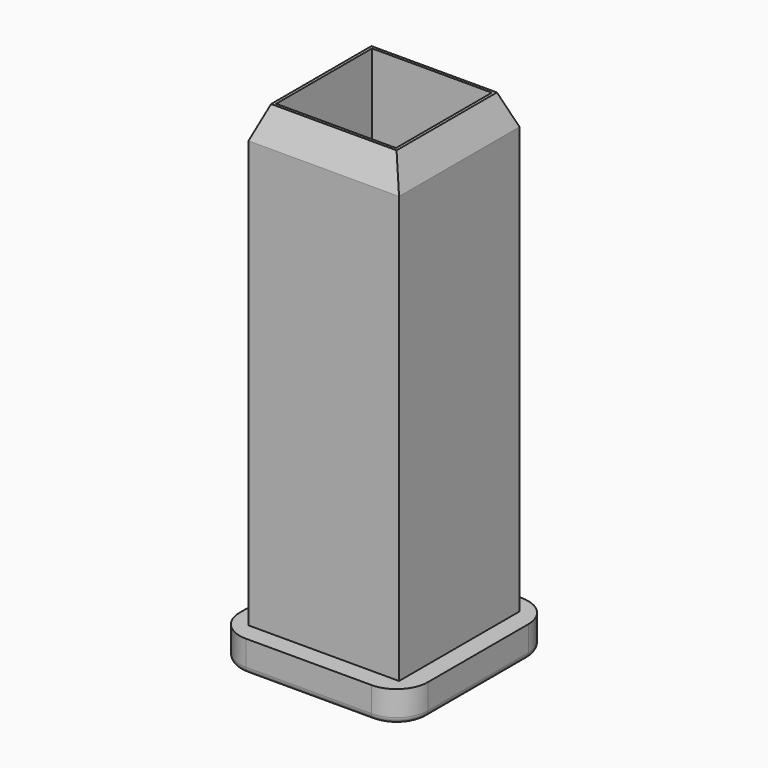
from build123d import *

# Parameters (mm, degrees)
F0_W         = 24
F0_H         = 24
F0_W_2       = 19.1
F0_H_2       = 19.1
F1_DEPTH     = 73
F2_W         = 30
F2_H         = 30
F2_W_2       = 19.1615689546
F2_H_2       = 19.1443199292
F3_DEPTH     = 5
F4_T4_DEPTH  = 19.1615689546
F4_T9_DEPTH  = 19.1443199292
F4_T14_DEPTH = 19.1615689546
F4_T19_DEPTH = 19.1443199292
F4_T25_DEPTH = 45.1428898176
F4_T30_DEPTH = 45.1256407922
F4_T38_DEPTH = 45.1428898176
F4_T43_DEPTH = 45.1256407922
F4_T51_DEPTH = 45.1428898176
F4_T56_DEPTH = 45.1256407922
F4_T64_DEPTH = 45.1256407922
F4_T69_DEPTH = 45.1428898176
F5_SIZE2     = 3
F5_SIZE      = 1
F6_R         = 5
F7_R         = 1
F8_SIZE2     = 2
F8_SIZE      = 5


# Not quite as in the source:
# - a fillet or chamfer that OpenCascade refuses, or shapes differently, is made with other operations: its cross-section is extruded or revolved along the edge and cut away or added


with BuildPart() as f1:
    # F0 (on Top) → F1 (new body)
    with BuildSketch(Plane.XY):
        with Locations((0.93195308, 1.8190721235)):
            Rectangle(F0_W, F0_H)
        with Locations((0.93195308, 1.8190721235)):
            Rectangle(F0_W_2, F0_H_2, mode=Mode.SUBTRACT)
    extrude(amount=F1_DEPTH)

    # F2 (on Top) → F3 (join)
    with BuildSketch(Plane.XY):
        with Locations((0.93195308, 1.8190721235)):
            Rectangle(F2_W, F2_H)
        with Locations((0.9246049449, 1.8198941834)):
            Rectangle(F2_W_2, F2_H_2, mode=Mode.SUBTRACT)
    extrude(amount=-F3_DEPTH)

    # F4: chamfer of 2 x 10 on 4 edges, made by hand


with BuildPart() as f4_tool2:
    # F4_s3 → F4_t4 (new body)
    with BuildSketch(Plane.YZ.offset(10.5053894222)):
        with BuildLine():
            Line((-9.8307122352, -5.3922322703), (-7.6738193271, 5.3922322703))
            Line((-7.6738193271, 5.3922322703), (-7.4738193271, 5.3922322703))
            ThreePointArc((-7.4738193271, 5.3922322703), (-7.5522657812, 0.1961161351), (-7.5522657812, -5))
            Line((-7.5522657812, -5), (-7.7522657812, -5.2))
            ThreePointArc((-7.7522657812, -5.2), (-8.7914890082, -5.2), (-9.8307122352, -5.5922322703))
            Line((-9.8307122352, -5.5922322703), (-9.8307122352, -5.3922322703))
        make_face()
    extrude(amount=-F4_T4_DEPTH)

    split(bisect_by=Plane.XY, keep=Keep.BOTTOM)


with BuildPart() as f1_1:
    add(f1.part)

    # F4_t1: cut F4_tool2
    add(f4_tool2.part, mode=Mode.SUBTRACT)


with BuildPart() as f4_tool7:
    # F4_s8 → F4_t9 (new body)
    with BuildSketch(Plane.XZ.offset(-11.392054148)):
        with BuildLine():
            Line((12.5838358762, -5.3922322703), (10.4269429681, 5.3922322703))
            Line((10.4269429681, 5.3922322703), (10.2269429681, 5.3922322703))
            ThreePointArc((10.2269429681, 5.3922322703), (10.3053894222, 0.1961161351), (10.3053894222, -5))
            Line((10.3053894222, -5), (10.5053894222, -5.2))
            ThreePointArc((10.5053894222, -5.2), (11.5446126492, -5.2), (12.5838358762, -5.5922322703))
            Line((12.5838358762, -5.5922322703), (12.5838358762, -5.3922322703))
        make_face()
    extrude(amount=F4_T9_DEPTH)

    split(bisect_by=Plane.XY, keep=Keep.BOTTOM)


with BuildPart() as f1_2:
    add(f1_1.part)

    # F4_t6: cut F4_tool7
    add(f4_tool7.part, mode=Mode.SUBTRACT)


with BuildPart() as f4_tool12:
    # F4_s13 → F4_t14 (new body)
    with BuildSketch(Plane.YZ.offset(-8.6561795324)):
        with BuildLine():
            Line((13.4705006021, -5.3922322703), (11.313607694, 5.3922322703))
            Line((11.313607694, 5.3922322703), (11.113607694, 5.3922322703))
            ThreePointArc((11.113607694, 5.3922322703), (11.192054148, 0.1961161351), (11.192054148, -5))
            Line((11.192054148, -5), (11.392054148, -5.2))
            ThreePointArc((11.392054148, -5.2), (12.431277375, -5.2), (13.4705006021, -5.5922322703))
            Line((13.4705006021, -5.5922322703), (13.4705006021, -5.3922322703))
        make_face()
    extrude(amount=F4_T14_DEPTH)

    split(bisect_by=Plane.XY, keep=Keep.BOTTOM)


with BuildPart() as f1_3:
    add(f1_2.part)

    # F4_t11: cut F4_tool12
    add(f4_tool12.part, mode=Mode.SUBTRACT)


with BuildPart() as f4_tool17:
    # F4_s18 → F4_t19 (new body)
    with BuildSketch(Plane.XZ.offset(7.7522657812)):
        with BuildLine():
            Line((-10.7346259865, -5.3922322703), (-8.5777330784, 5.3922322703))
            Line((-8.5777330784, 5.3922322703), (-8.3777330784, 5.3922322703))
            ThreePointArc((-8.3777330784, 5.3922322703), (-8.4561795324, 0.1961161351), (-8.4561795324, -5))
            Line((-8.4561795324, -5), (-8.6561795324, -5.2))
            ThreePointArc((-8.6561795324, -5.2), (-9.6954027594, -5.2), (-10.7346259865, -5.5922322703))
            Line((-10.7346259865, -5.5922322703), (-10.7346259865, -5.3922322703))
        make_face()
    extrude(amount=-F4_T19_DEPTH)

    split(bisect_by=Plane.XY, keep=Keep.BOTTOM)


with BuildPart() as f1_4:
    add(f1_3.part)

    # F4_t16: cut F4_tool17
    add(f4_tool17.part, mode=Mode.SUBTRACT)


with BuildPart() as f4_tool23:
    # F4_s24 → F4_t25 (new body)
    with BuildSketch(Plane.YZ.offset(36.4867102851)):
        with BuildLine():
            Line((-9.8307122352, -5.3922322703), (-7.6738193271, 5.3922322703))
            Line((-7.6738193271, 5.3922322703), (-7.4738193271, 5.3922322703))
            ThreePointArc((-7.4738193271, 5.3922322703), (-7.5522657812, 0.1961161351), (-7.5522657812, -5))
            Line((-7.5522657812, -5), (-7.7522657812, -5.2))
            ThreePointArc((-7.7522657812, -5.2), (-8.7914890082, -5.2), (-9.8307122352, -5.5922322703))
            Line((-9.8307122352, -5.5922322703), (-9.8307122352, -5.3922322703))
        make_face()
    extrude(amount=-F4_T25_DEPTH)

    split(bisect_by=Plane.XY, keep=Keep.BOTTOM)

    split(bisect_by=Plane.YZ.offset(10.5053894222), keep=Keep.TOP)


with BuildPart() as f4_tool28:
    # F4_s29 → F4_t30 (new body)
    with BuildSketch(Plane.XZ.offset(-11.392054148)):
        with BuildLine():
            Line((12.5838358762, -5.3922322703), (10.4269429681, 5.3922322703))
            Line((10.4269429681, 5.3922322703), (10.2269429681, 5.3922322703))
            ThreePointArc((10.2269429681, 5.3922322703), (10.3053894222, 0.1961161351), (10.3053894222, -5))
            Line((10.3053894222, -5), (10.5053894222, -5.2))
            ThreePointArc((10.5053894222, -5.2), (11.5446126492, -5.2), (12.5838358762, -5.5922322703))
            Line((12.5838358762, -5.5922322703), (12.5838358762, -5.3922322703))
        make_face()
    extrude(amount=F4_T30_DEPTH)

    split(bisect_by=Plane.XY, keep=Keep.BOTTOM)

    split(bisect_by=Plane.XZ.offset(7.7522657812), keep=Keep.TOP)


with BuildPart() as f4_tool23_1:
    add(f4_tool23.part)

    # F4_t33: intersect F4_tool28
    add(f4_tool28.part, mode=Mode.INTERSECT)


with BuildPart() as f1_5:
    add(f1_4.part)

    # F4_t21: cut F4_tool23
    add(f4_tool23_1.part, mode=Mode.SUBTRACT)


with BuildPart() as f4_tool36:
    # F4_s37 → F4_t38 (new body)
    with BuildSketch(Plane.YZ.offset(10.5053894222)):
        with BuildLine():
            Line((-9.8307122352, -5.3922322703), (-7.6738193271, 5.3922322703))
            Line((-7.6738193271, 5.3922322703), (-7.4738193271, 5.3922322703))
            ThreePointArc((-7.4738193271, 5.3922322703), (-7.5522657812, 0.1961161351), (-7.5522657812, -5))
            Line((-7.5522657812, -5), (-7.7522657812, -5.2))
            ThreePointArc((-7.7522657812, -5.2), (-8.7914890082, -5.2), (-9.8307122352, -5.5922322703))
            Line((-9.8307122352, -5.5922322703), (-9.8307122352, -5.3922322703))
        make_face()
    extrude(amount=-F4_T38_DEPTH)

    split(bisect_by=Plane.XY, keep=Keep.BOTTOM)

    split(bisect_by=Plane.YZ.offset(-8.6561795324), keep=Keep.BOTTOM)


with BuildPart() as f4_tool41:
    # F4_s42 → F4_t43 (new body)
    with BuildSketch(Plane.XZ.offset(33.7335866441)):
        with BuildLine():
            Line((-10.7346259865, -5.3922322703), (-8.5777330784, 5.3922322703))
            Line((-8.5777330784, 5.3922322703), (-8.3777330784, 5.3922322703))
            ThreePointArc((-8.3777330784, 5.3922322703), (-8.4561795324, 0.1961161351), (-8.4561795324, -5))
            Line((-8.4561795324, -5), (-8.6561795324, -5.2))
            ThreePointArc((-8.6561795324, -5.2), (-9.6954027594, -5.2), (-10.7346259865, -5.5922322703))
            Line((-10.7346259865, -5.5922322703), (-10.7346259865, -5.3922322703))
        make_face()
    extrude(amount=-F4_T43_DEPTH)

    split(bisect_by=Plane.XY, keep=Keep.BOTTOM)

    split(bisect_by=Plane.XZ.offset(7.7522657812), keep=Keep.TOP)


with BuildPart() as f4_tool36_1:
    add(f4_tool36.part)

    # F4_t46: intersect F4_tool41
    add(f4_tool41.part, mode=Mode.INTERSECT)


with BuildPart() as f1_6:
    add(f1_5.part)

    # F4_t34: cut F4_tool36
    add(f4_tool36_1.part, mode=Mode.SUBTRACT)


with BuildPart() as f4_tool49:
    # F4_s50 → F4_t51 (new body)
    with BuildSketch(Plane.YZ.offset(-8.6561795324)):
        with BuildLine():
            Line((13.4705006021, -5.3922322703), (11.313607694, 5.3922322703))
            Line((11.313607694, 5.3922322703), (11.113607694, 5.3922322703))
            ThreePointArc((11.113607694, 5.3922322703), (11.192054148, 0.1961161351), (11.192054148, -5))
            Line((11.192054148, -5), (11.392054148, -5.2))
            ThreePointArc((11.392054148, -5.2), (12.431277375, -5.2), (13.4705006021, -5.5922322703))
            Line((13.4705006021, -5.5922322703), (13.4705006021, -5.3922322703))
        make_face()
    extrude(amount=F4_T51_DEPTH)

    split(bisect_by=Plane.XY, keep=Keep.BOTTOM)

    split(bisect_by=Plane.YZ.offset(10.5053894222), keep=Keep.TOP)


with BuildPart() as f4_tool54:
    # F4_s55 → F4_t56 (new body)
    with BuildSketch(Plane.XZ.offset(-37.373375011)):
        with BuildLine():
            Line((12.5838358762, -5.3922322703), (10.4269429681, 5.3922322703))
            Line((10.4269429681, 5.3922322703), (10.2269429681, 5.3922322703))
            ThreePointArc((10.2269429681, 5.3922322703), (10.3053894222, 0.1961161351), (10.3053894222, -5))
            Line((10.3053894222, -5), (10.5053894222, -5.2))
            ThreePointArc((10.5053894222, -5.2), (11.5446126492, -5.2), (12.5838358762, -5.5922322703))
            Line((12.5838358762, -5.5922322703), (12.5838358762, -5.3922322703))
        make_face()
    extrude(amount=F4_T56_DEPTH)

    split(bisect_by=Plane.XY, keep=Keep.BOTTOM)

    split(bisect_by=Plane.XZ.offset(-11.392054148), keep=Keep.BOTTOM)


with BuildPart() as f4_tool49_1:
    add(f4_tool49.part)

    # F4_t59: intersect F4_tool54
    add(f4_tool54.part, mode=Mode.INTERSECT)


with BuildPart() as f1_7:
    add(f1_6.part)

    # F4_t47: cut F4_tool49
    add(f4_tool49_1.part, mode=Mode.SUBTRACT)


with BuildPart() as f4_tool62:
    # F4_s63 → F4_t64 (new body)
    with BuildSketch(Plane.XZ.offset(7.7522657812)):
        with BuildLine():
            Line((-10.7346259865, -5.3922322703), (-8.5777330784, 5.3922322703))
            Line((-8.5777330784, 5.3922322703), (-8.3777330784, 5.3922322703))
            ThreePointArc((-8.3777330784, 5.3922322703), (-8.4561795324, 0.1961161351), (-8.4561795324, -5))
            Line((-8.4561795324, -5), (-8.6561795324, -5.2))
            ThreePointArc((-8.6561795324, -5.2), (-9.6954027594, -5.2), (-10.7346259865, -5.5922322703))
            Line((-10.7346259865, -5.5922322703), (-10.7346259865, -5.3922322703))
        make_face()
    extrude(amount=-F4_T64_DEPTH)

    split(bisect_by=Plane.XY, keep=Keep.BOTTOM)

    split(bisect_by=Plane.XZ.offset(-11.392054148), keep=Keep.BOTTOM)


with BuildPart() as f4_tool67:
    # F4_s68 → F4_t69 (new body)
    with BuildSketch(Plane.YZ.offset(-34.6375003954)):
        with BuildLine():
            Line((13.4705006021, -5.3922322703), (11.313607694, 5.3922322703))
            Line((11.313607694, 5.3922322703), (11.113607694, 5.3922322703))
            ThreePointArc((11.113607694, 5.3922322703), (11.192054148, 0.1961161351), (11.192054148, -5))
            Line((11.192054148, -5), (11.392054148, -5.2))
            ThreePointArc((11.392054148, -5.2), (12.431277375, -5.2), (13.4705006021, -5.5922322703))
            Line((13.4705006021, -5.5922322703), (13.4705006021, -5.3922322703))
        make_face()
    extrude(amount=F4_T69_DEPTH)

    split(bisect_by=Plane.XY, keep=Keep.BOTTOM)

    split(bisect_by=Plane.YZ.offset(-8.6561795324), keep=Keep.BOTTOM)


with BuildPart() as f4_tool62_1:
    add(f4_tool62.part)

    # F4_t72: intersect F4_tool67
    add(f4_tool67.part, mode=Mode.INTERSECT)


with BuildPart() as f1_8:
    add(f1_7.part)

    # F4_t60: cut F4_tool62
    add(f4_tool62_1.part, mode=Mode.SUBTRACT)

    # F5
    f5_edges = [f1_8.edges().sort_by_distance(p)[0] for p in [
        (0.931953, -7.730928, 0),
        (10.481953, 1.819072, 0),
        (0.931953, 11.369072, 0),
        (-8.618047, 1.819072, 0),
    ]]
    f5_side = f1_8.faces().sort_by_distance((0.931953, 11.66822, 0))[0]
    chamfer(f5_edges, length=F5_SIZE, length2=F5_SIZE2, reference=f5_side)

    # F6
    f6_edges = [f1_8.edges().sort_by_distance(p)[0] for p in [
        (-14.068047, 16.819072, -2.5),
        (15.931953, 16.819072, -2.5),
        (15.931953, -13.180928, -2.5),
        (-14.068047, -13.180928, -2.5),
    ]]
    fillet(f6_edges, radius=F6_R)

    # F7
    f7_edges = [f1_8.edges().sort_by_distance(p)[0] for p in [
        (15.931953, 1.819072, -5),
        (14.467487, -11.716462, -5),
        (0.931953, -13.180928, -5),
        (-14.068047, 1.819072, -5),
        (-12.603581, 15.354606, -5),
        (-12.603581, -11.716462, -5),
        (0.931953, 16.819072, -5),
        (14.467487, 15.354606, -5),
    ]]
    fillet(f7_edges, radius=F7_R)

    # F8
    f8_edges = [f1_8.edges().sort_by_distance(p)[0] for p in [
        (0.931953, 13.819072, 73),
        (12.931953, 1.819072, 73),
        (0.931953, -10.180928, 73),
        (-11.068047, 1.819072, 73),
    ]]
    chamfer(f8_edges, length=F8_SIZE, length2=F8_SIZE2)


solid = f1_8.part
